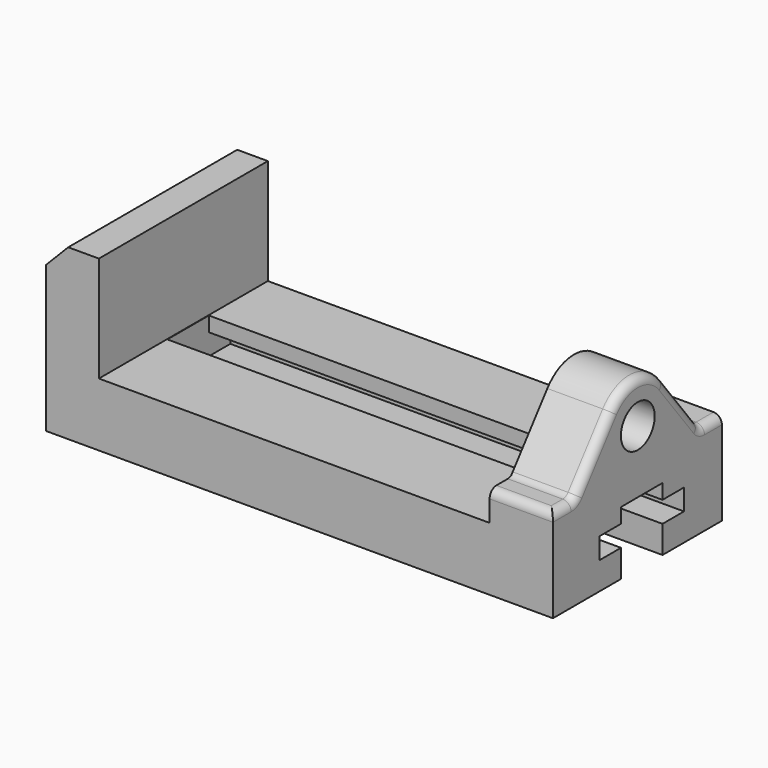
from build123d import *

# Parameters (mm, degrees)
F1_DEPTH = 127
F3_DEPTH = 38.354
F4_R     = 12.7
F5_DEPTH = 63.5
F7_DEPTH = 272.796
F8_R     = 5.08


with BuildPart() as f1:
    # F0 (on Front) → F1 (new body)
    with BuildSketch(Plane.XZ):
        Polygon((0, 87.987836793), (0, 0), (304.8, 0), (304.8, 55.88), (266.7, 55.88), (266.7, 38.1), (31.75, 38.1), (31.75, 101.6), (13.3270969392, 101.6), align=None)
    extrude(amount=F1_DEPTH)

    # F2 (on face) → F3 (join)
    with BuildSketch(Plane.YZ.offset(304.8)):
        with BuildLine():
            Line((-83.2950948956, 91.4038064892), (-110.8501477266, 55.88))
            Line((-110.8501477266, 55.88), (-15.6001477266, 55.88))
            Line((-15.6001477266, 55.88), (-43.1552005575, 91.4038064892))
            ThreePointArc((-43.1552005575, 91.4038064892), (-63.2251477266, 101.2359800311), (-83.2950948956, 91.4038064892))
        make_face()
    extrude(amount=-F3_DEPTH)

    # F4 (on face) → F5 (cut, symmetric)
    with BuildSketch(Plane.YZ.offset(304.8)):
        with Locations((-63.2251477266, 75.8359800311)):
            Circle(F4_R)
    extrude(amount=F5_DEPTH, both=True, mode=Mode.SUBTRACT)

    # F6 (on face) → F7 (cut)
    with BuildSketch(Plane.YZ.offset(304.8)):
        Polygon((-75.8447764756, 16.51), (-75.8447764756, 0), (-44.662312481, 0), (-44.662312481, 16.51), (-28.5035444783, 16.51), (-28.5035444783, 29.21), (-44.662312481, 29.21), (-44.662312481, 38.1537896351), (-75.8601041585, 38.1), (-75.8447764756, 29.21), (-92.0035444783, 29.21), (-92.0035444783, 16.51), align=None)
    extrude(amount=-F7_DEPTH, mode=Mode.SUBTRACT)

    # F8
    f8_edges = [f1.edges().sort_by_distance(p)[0] for p in [
        (304.8, -97.072621, 73.641903),
        (304.8, -7.800074, 55.88),
        (304.8, -118.925074, 55.88),
        (285.75, -127, 55.88),
        (285.623, -83.295095, 91.403806),
        (285.623, -43.155201, 91.403806),
        (304.8, -29.377674, 73.641903),
        (304.8, -63.225148, 101.23598),
        (285.75, -15.600148, 55.88),
        (285.75, -110.850148, 55.88),
    ]]
    fillet(f8_edges, radius=F8_R)


solid = f1.part
